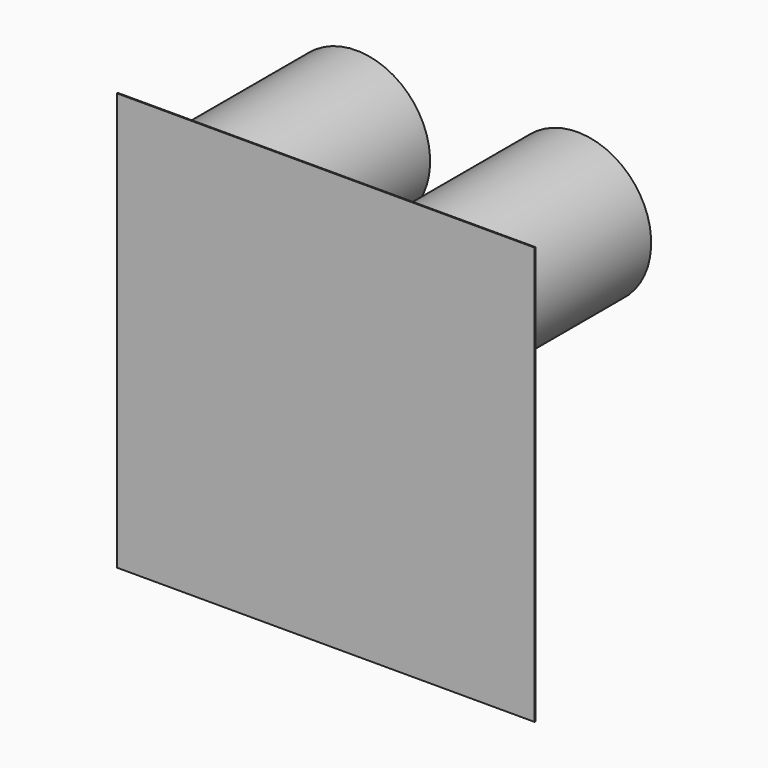
from build123d import *

# Parameters (mm, degrees)
F0_W     = 10000
F0_H     = 10000
F1_DEPTH = 25
F2_R     = 1764.5
F3_DEPTH = 4572


# Not quite as in the source:
# - a feature names something its author has since deleted; it is built from what else it names


with BuildPart() as f1:
    # F0 (on Front) → F1 (new body)
    with BuildSketch(Plane.XZ):
        with Locations((-5000, 5000)):
            Rectangle(F0_W, F0_H)
    extrude(amount=F1_DEPTH)

    # F2 (on face) → F3 (join)
    with BuildSketch(Plane(origin=(0, 0, 0), x_dir=(-1, 0, 0), z_dir=(0, 1, 0))):
        with Locations((2648, 7942)):
            Circle(F2_R)
        with Locations((7942, 7942)):
            Circle(F2_R)
    extrude(amount=F3_DEPTH)


solid = f1.part
